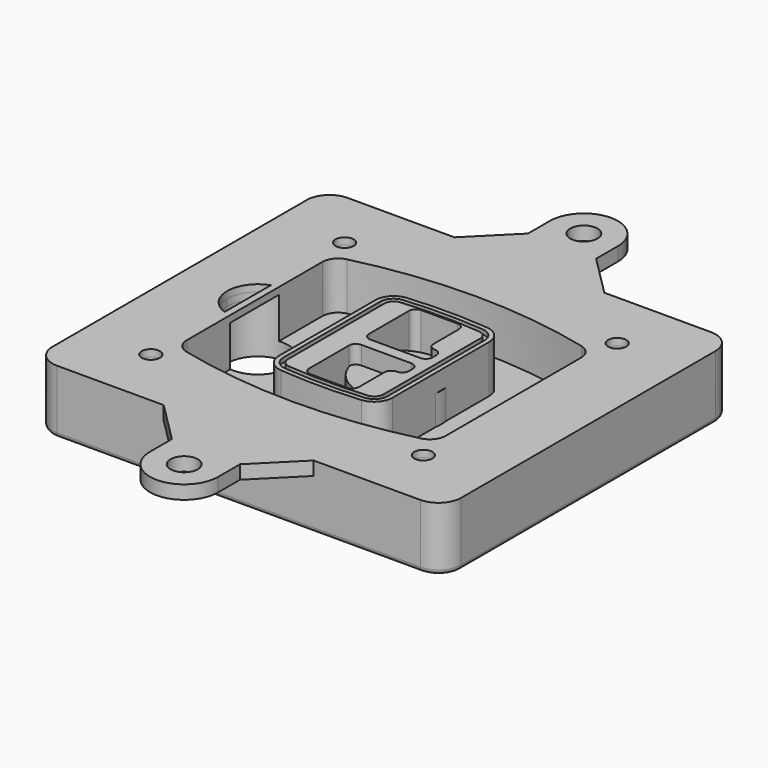
from build123d import *

# Parameters (mm, degrees)
F0_R      = 4
F1_DEPTH  = 25
F2_DEPTH  = 3
F3_DEPTH  = 18
F5_DEPTH  = 21
F6_DEPTH  = 2
F8_DEPTH  = 20
F9_DEPTH  = 16
F10_DEPTH = 25
F7_R      = 6
F7_R_2    = 4
F11_DEPTH = 6
F13_DEPTH = 9
F15_R     = 2
F16_R     = 6
F16_R_2   = 4
F17_DEPTH = 3


# Not quite as in the source:
# - a feature of the source that left no trace in its solid (it failed there, or was rolled back) is left out
# - a feature names something its author has since deleted; it is built from what else it names


with BuildPart() as f1:
    # F0 (on Top) → F1 (new body)
    with BuildSketch(Plane.XY):
        with BuildLine():
            ThreePointArc((-90, -70), (-87.0710678119, -77.0710678119), (-80, -80))
            Line((-80, -80), (80, -80))
            ThreePointArc((80, -80), (87.0710678119, -77.0710678119), (90, -70))
            Line((90, -70), (90, 70))
            ThreePointArc((90, 70), (87.0710678119, 77.0710678119), (80, 80))
            Line((80, 80), (-80, 80))
            ThreePointArc((-80, 80), (-87.0710678119, 77.0710678119), (-90, 70))
            Line((-90, 70), (-90, -70))
        make_face()
        with Locations((-60, -53.3333333333)):
            Circle(F0_R, mode=Mode.SUBTRACT)
        with Locations((60, -53.3333333333)):
            Circle(F0_R, mode=Mode.SUBTRACT)
        with Locations((-60, 53.3333333333)):
            Circle(F0_R, mode=Mode.SUBTRACT)
        with BuildLine():
            ThreePointArc((-64, 37.2990447398), (-61.0143011354, 45.9411029726), (-53.3306899286, 50.8970778549))
            ThreePointArc((-53.3306899286, 50.8970778549), (0, 57.3333333333), (53.3306899286, 50.8970778549))
            ThreePointArc((53.3306899286, 50.8970778549), (61.0143011354, 45.9411029726), (64, 37.2990447398))
            Line((64, 37.2990447398), (64, -37.2990447398))
            ThreePointArc((64, -37.2990447398), (61.0143011354, -45.9411029726), (53.3306899286, -50.8970778549))
            ThreePointArc((53.3306899286, -50.8970778549), (0, -57.3333333333), (-53.3306899286, -50.8970778549))
            ThreePointArc((-53.3306899286, -50.8970778549), (-61.0143011354, -45.9411029726), (-64, -37.2990447398))
            Line((-64, -37.2990447398), (-64, 37.2990447398))
        make_face(mode=Mode.SUBTRACT)
        with Locations((60, 53.3333333333)):
            Circle(F0_R, mode=Mode.SUBTRACT)
        with BuildLine():
            ThreePointArc((53.3306899286, 50.8970778549), (0, 57.3333333333), (-53.3306899286, 50.8970778549))
            ThreePointArc((-53.3306899286, 50.8970778549), (-61.0143011354, 45.9411029726), (-64, 37.2990447398))
            Line((-64, 37.2990447398), (-64, -37.2990447398))
            ThreePointArc((-64, -37.2990447398), (-61.0143011354, -45.9411029726), (-53.3306899286, -50.8970778549))
            ThreePointArc((-53.3306899286, -50.8970778549), (0, -57.3333333333), (53.3306899286, -50.8970778549))
            ThreePointArc((53.3306899286, -50.8970778549), (61.0143011354, -45.9411029726), (64, -37.2990447398))
            Line((64, -37.2990447398), (64, 37.2990447398))
            ThreePointArc((64, 37.2990447398), (61.0143011354, 45.9411029726), (53.3306899286, 50.8970778549))
        make_face()
        with BuildLine():
            Line((-60, -37.2990447398), (-60, 37.2990447398))
            ThreePointArc((-60, 37.2990447398), (-57.8673579538, 43.4719434775), (-52.3790642347, 47.0119255363))
            ThreePointArc((-52.3790642347, 47.0119255363), (0, 53.3333333333), (52.3790642347, 47.0119255363))
            ThreePointArc((52.3790642347, 47.0119255363), (57.8673579538, 43.4719434775), (60, 37.2990447398))
            Line((60, 37.2990447398), (60, -37.2990447398))
            ThreePointArc((60, -37.2990447398), (57.8673579538, -43.4719434775), (52.3790642347, -47.0119255363))
            ThreePointArc((52.3790642347, -47.0119255363), (0, -53.3333333333), (-52.3790642347, -47.0119255363))
            ThreePointArc((-52.3790642347, -47.0119255363), (-57.8673579538, -43.4719434775), (-60, -37.2990447398))
        make_face(mode=Mode.SUBTRACT)
        with BuildLine():
            ThreePointArc((-52.3790642347, 47.0119255363), (-57.8673579538, 43.4719434775), (-60, 37.2990447398))
            Line((-60, 37.2990447398), (-60, -37.2990447398))
            ThreePointArc((-60, -37.2990447398), (-57.8673579538, -43.4719434775), (-52.3790642347, -47.0119255363))
            ThreePointArc((-52.3790642347, -47.0119255363), (0, -53.3333333333), (52.3790642347, -47.0119255363))
            ThreePointArc((52.3790642347, -47.0119255363), (57.8673579538, -43.4719434775), (60, -37.2990447398))
            Line((60, -37.2990447398), (60, 37.2990447398))
            ThreePointArc((60, 37.2990447398), (57.8673579538, 43.4719434775), (52.3790642347, 47.0119255363))
            ThreePointArc((52.3790642347, 47.0119255363), (0, 53.3333333333), (-52.3790642347, 47.0119255363))
        make_face()
        with BuildLine():
            ThreePointArc((51.6653449643, 44.0980612973), (55.5071505677, 41.6200738562), (57, 37.2990447398))
            Line((57, 37.2990447398), (57, -37.2990447398))
            ThreePointArc((57, -37.2990447398), (55.5071505677, -41.6200738562), (51.6653449643, -44.0980612973))
            ThreePointArc((51.6653449643, -44.0980612973), (0, -50.3333333333), (-51.6653449643, -44.0980612973))
            ThreePointArc((-51.6653449643, -44.0980612973), (-55.5071505677, -41.6200738562), (-57, -37.2990447398))
            Line((-57, -37.2990447398), (-57, 37.2990447398))
            ThreePointArc((-57, 37.2990447398), (-55.5071505677, 41.6200738562), (-51.6653449643, 44.0980612973))
            ThreePointArc((-51.6653449643, 44.0980612973), (0, 50.3333333333), (51.6653449643, 44.0980612973))
        make_face(mode=Mode.SUBTRACT)
        with BuildLine():
            Line((57, -37.2990447398), (57, 37.2990447398))
            ThreePointArc((57, 37.2990447398), (55.5071505677, 41.6200738562), (51.6653449643, 44.0980612973))
            ThreePointArc((51.6653449643, 44.0980612973), (0, 50.3333333333), (-51.6653449643, 44.0980612973))
            ThreePointArc((-51.6653449643, 44.0980612973), (-55.5071505677, 41.6200738562), (-57, 37.2990447398))
            Line((-57, 37.2990447398), (-57, -37.2990447398))
            ThreePointArc((-57, -37.2990447398), (-55.5071505677, -41.6200738562), (-51.6653449643, -44.0980612973))
            ThreePointArc((-51.6653449643, -44.0980612973), (0, -50.3333333333), (51.6653449643, -44.0980612973))
            ThreePointArc((51.6653449643, -44.0980612973), (55.5071505677, -41.6200738562), (57, -37.2990447398))
        make_face()
    extrude(amount=-F1_DEPTH)

    # F0 (on Top) → F2 (join)
    with BuildSketch(Plane.XY):
        with BuildLine():
            ThreePointArc((-52.3790642347, 47.0119255363), (-57.8673579538, 43.4719434775), (-60, 37.2990447398))
            Line((-60, 37.2990447398), (-60, -37.2990447398))
            ThreePointArc((-60, -37.2990447398), (-57.8673579538, -43.4719434775), (-52.3790642347, -47.0119255363))
            ThreePointArc((-52.3790642347, -47.0119255363), (0, -53.3333333333), (52.3790642347, -47.0119255363))
            ThreePointArc((52.3790642347, -47.0119255363), (57.8673579538, -43.4719434775), (60, -37.2990447398))
            Line((60, -37.2990447398), (60, 37.2990447398))
            ThreePointArc((60, 37.2990447398), (57.8673579538, 43.4719434775), (52.3790642347, 47.0119255363))
            ThreePointArc((52.3790642347, 47.0119255363), (0, 53.3333333333), (-52.3790642347, 47.0119255363))
        make_face()
        with BuildLine():
            ThreePointArc((51.6653449643, 44.0980612973), (55.5071505677, 41.6200738562), (57, 37.2990447398))
            Line((57, 37.2990447398), (57, -37.2990447398))
            ThreePointArc((57, -37.2990447398), (55.5071505677, -41.6200738562), (51.6653449643, -44.0980612973))
            ThreePointArc((51.6653449643, -44.0980612973), (0, -50.3333333333), (-51.6653449643, -44.0980612973))
            ThreePointArc((-51.6653449643, -44.0980612973), (-55.5071505677, -41.6200738562), (-57, -37.2990447398))
            Line((-57, -37.2990447398), (-57, 37.2990447398))
            ThreePointArc((-57, 37.2990447398), (-55.5071505677, 41.6200738562), (-51.6653449643, 44.0980612973))
            ThreePointArc((-51.6653449643, 44.0980612973), (0, 50.3333333333), (51.6653449643, 44.0980612973))
        make_face(mode=Mode.SUBTRACT)
    extrude(amount=F2_DEPTH)

    # F0 (on Top) → F3 (cut)
    with BuildSketch(Plane.XY):
        with BuildLine():
            Line((57, -37.2990447398), (57, 37.2990447398))
            ThreePointArc((57, 37.2990447398), (55.5071505677, 41.6200738562), (51.6653449643, 44.0980612973))
            ThreePointArc((51.6653449643, 44.0980612973), (0, 50.3333333333), (-51.6653449643, 44.0980612973))
            ThreePointArc((-51.6653449643, 44.0980612973), (-55.5071505677, 41.6200738562), (-57, 37.2990447398))
            Line((-57, 37.2990447398), (-57, -37.2990447398))
            ThreePointArc((-57, -37.2990447398), (-55.5071505677, -41.6200738562), (-51.6653449643, -44.0980612973))
            ThreePointArc((-51.6653449643, -44.0980612973), (0, -50.3333333333), (51.6653449643, -44.0980612973))
            ThreePointArc((51.6653449643, -44.0980612973), (55.5071505677, -41.6200738562), (57, -37.2990447398))
        make_face()
    extrude(amount=-F3_DEPTH, mode=Mode.SUBTRACT)

    # F4 (on face) → F5 (join, through all)
    with BuildSketch(Plane.XY.offset(3)):
        with BuildLine():
            ThreePointArc((-25, -26.587695628), (-22.8992979869, -31.9912392117), (-17.7004291845, -34.5569740744))
            ThreePointArc((-17.7004291845, -34.5569740744), (0, -35.3333333333), (17.7004291845, -34.5569740744))
            ThreePointArc((17.7004291845, -34.5569740744), (22.8992979869, -31.9912392117), (25, -26.587695628))
            Line((25, -26.587695628), (25, 26.587695628))
            ThreePointArc((25, 26.587695628), (22.8992979869, 31.9912392117), (17.7004291845, 34.5569740744))
            ThreePointArc((17.7004291845, 34.5569740744), (0, 35.3333333333), (-17.7004291845, 34.5569740744))
            ThreePointArc((-17.7004291845, 34.5569740744), (-22.8992979869, 31.9912392117), (-25, 26.587695628))
            Line((-25, 26.587695628), (-25, -26.587695628))
        make_face()
        with BuildLine():
            ThreePointArc((17.5253218884, 32.5646544628), (21.4244734902, 30.6403533158), (23, 26.587695628))
            Line((23, 26.587695628), (23, -26.587695628))
            ThreePointArc((23, -26.587695628), (21.4244734902, -30.6403533158), (17.5253218884, -32.5646544628))
            ThreePointArc((17.5253218884, -32.5646544628), (0, -33.3333333333), (-17.5253218884, -32.5646544628))
            ThreePointArc((-17.5253218884, -32.5646544628), (-21.4244734902, -30.6403533158), (-23, -26.587695628))
            Line((-23, -26.587695628), (-23, 26.587695628))
            ThreePointArc((-23, 26.587695628), (-21.4244734902, 30.6403533158), (-17.5253218884, 32.5646544628))
            ThreePointArc((-17.5253218884, 32.5646544628), (0, 33.3333333333), (17.5253218884, 32.5646544628))
        make_face(mode=Mode.SUBTRACT)
        with BuildLine():
            Line((23, -26.587695628), (23, 26.587695628))
            ThreePointArc((23, 26.587695628), (21.4244734902, 30.6403533158), (17.5253218884, 32.5646544628))
            ThreePointArc((17.5253218884, 32.5646544628), (0, 33.3333333333), (-17.5253218884, 32.5646544628))
            ThreePointArc((-17.5253218884, 32.5646544628), (-21.4244734902, 30.6403533158), (-23, 26.587695628))
            Line((-23, 26.587695628), (-23, -26.587695628))
            ThreePointArc((-23, -26.587695628), (-21.4244734902, -30.6403533158), (-17.5253218884, -32.5646544628))
            ThreePointArc((-17.5253218884, -32.5646544628), (0, -33.3333333333), (17.5253218884, -32.5646544628))
            ThreePointArc((17.5253218884, -32.5646544628), (21.4244734902, -30.6403533158), (23, -26.587695628))
        make_face()
        with BuildLine():
            ThreePointArc((17.3502145923, 30.5723348512), (19.9496489934, 29.2894674198), (21, 26.587695628))
            Line((21, 26.587695628), (21, -26.587695628))
            ThreePointArc((21, -26.587695628), (19.9496489934, -29.2894674198), (17.3502145923, -30.5723348512))
            ThreePointArc((17.3502145923, -30.5723348512), (0, -31.3333333333), (-17.3502145923, -30.5723348512))
            ThreePointArc((-17.3502145923, -30.5723348512), (-19.9496489934, -29.2894674198), (-21, -26.587695628))
            Line((-21, -26.587695628), (-21, 26.587695628))
            ThreePointArc((-21, 26.587695628), (-19.9496489934, 29.2894674198), (-17.3502145923, 30.5723348512))
            ThreePointArc((-17.3502145923, 30.5723348512), (0, 31.3333333333), (17.3502145923, 30.5723348512))
        make_face(mode=Mode.SUBTRACT)
        with BuildLine():
            Line((21, -26.587695628), (21, 26.587695628))
            ThreePointArc((21, 26.587695628), (19.9496489934, 29.2894674198), (17.3502145923, 30.5723348512))
            ThreePointArc((17.3502145923, 30.5723348512), (0, 31.3333333333), (-17.3502145923, 30.5723348512))
            ThreePointArc((-17.3502145923, 30.5723348512), (-19.9496489934, 29.2894674198), (-21, 26.587695628))
            Line((-21, 26.587695628), (-21, -26.587695628))
            ThreePointArc((-21, -26.587695628), (-19.9496489934, -29.2894674198), (-17.3502145923, -30.5723348512))
            ThreePointArc((-17.3502145923, -30.5723348512), (0, -31.3333333333), (17.3502145923, -30.5723348512))
            ThreePointArc((17.3502145923, -30.5723348512), (19.9496489934, -29.2894674198), (21, -26.587695628))
        make_face()
        with BuildLine():
            Line((-8, -2.5), (14, -2.5))
            ThreePointArc((14, -2.5), (16.1213203436, -3.3786796564), (17, -5.5))
            Line((17, -5.5), (17, -7.5))
            ThreePointArc((17, -7.5), (16.1213203436, -9.6213203436), (14, -10.5))
            ThreePointArc((14, -10.5), (11.8786796564, -11.3786796564), (11, -13.5))
            Line((11, -13.5), (11, -27.5))
            ThreePointArc((11, -27.5), (10.1213203436, -29.6213203436), (8, -30.5))
            Line((8, -30.5), (-8, -30.5))
            ThreePointArc((-8, -30.5), (-10.1213203436, -29.6213203436), (-11, -27.5))
            Line((-11, -27.5), (-11, -5.5))
            ThreePointArc((-11, -5.5), (-10.1213203436, -3.3786796564), (-8, -2.5))
        make_face(mode=Mode.SUBTRACT)
        with BuildLine():
            ThreePointArc((-8, 2.5), (-10.1213203436, 3.3786796564), (-11, 5.5))
            Line((-11, 5.5), (-11, 27.5))
            ThreePointArc((-11, 27.5), (-10.1213203436, 29.6213203436), (-8, 30.5))
            Line((-8, 30.5), (8, 30.5))
            ThreePointArc((8, 30.5), (10.1213203436, 29.6213203436), (11, 27.5))
            Line((11, 27.5), (11, 13.5))
            ThreePointArc((11, 13.5), (11.8786796564, 11.3786796564), (14, 10.5))
            ThreePointArc((14, 10.5), (16.1213203436, 9.6213203436), (17, 7.5))
            Line((17, 7.5), (17, 5.5))
            ThreePointArc((17, 5.5), (16.1213203436, 3.3786796564), (14, 2.5))
            Line((14, 2.5), (-8, 2.5))
        make_face(mode=Mode.SUBTRACT)
    extrude(amount=-F5_DEPTH)

    # F4 (on face) → F6 (cut)
    with BuildSketch(Plane.XY.offset(3)):
        with BuildLine():
            Line((23, -26.587695628), (23, 26.587695628))
            ThreePointArc((23, 26.587695628), (21.4244734902, 30.6403533158), (17.5253218884, 32.5646544628))
            ThreePointArc((17.5253218884, 32.5646544628), (0, 33.3333333333), (-17.5253218884, 32.5646544628))
            ThreePointArc((-17.5253218884, 32.5646544628), (-21.4244734902, 30.6403533158), (-23, 26.587695628))
            Line((-23, 26.587695628), (-23, -26.587695628))
            ThreePointArc((-23, -26.587695628), (-21.4244734902, -30.6403533158), (-17.5253218884, -32.5646544628))
            ThreePointArc((-17.5253218884, -32.5646544628), (0, -33.3333333333), (17.5253218884, -32.5646544628))
            ThreePointArc((17.5253218884, -32.5646544628), (21.4244734902, -30.6403533158), (23, -26.587695628))
        make_face()
        with BuildLine():
            ThreePointArc((17.3502145923, 30.5723348512), (19.9496489934, 29.2894674198), (21, 26.587695628))
            Line((21, 26.587695628), (21, -26.587695628))
            ThreePointArc((21, -26.587695628), (19.9496489934, -29.2894674198), (17.3502145923, -30.5723348512))
            ThreePointArc((17.3502145923, -30.5723348512), (0, -31.3333333333), (-17.3502145923, -30.5723348512))
            ThreePointArc((-17.3502145923, -30.5723348512), (-19.9496489934, -29.2894674198), (-21, -26.587695628))
            Line((-21, -26.587695628), (-21, 26.587695628))
            ThreePointArc((-21, 26.587695628), (-19.9496489934, 29.2894674198), (-17.3502145923, 30.5723348512))
            ThreePointArc((-17.3502145923, 30.5723348512), (0, 31.3333333333), (17.3502145923, 30.5723348512))
        make_face(mode=Mode.SUBTRACT)
    extrude(amount=-F6_DEPTH, mode=Mode.SUBTRACT)

    # F7 (on face) → F8 (join)
    with BuildSketch(Plane(origin=(0, 0, -25), x_dir=(1, 0, 0), z_dir=(0, 0, -1))):
        with BuildLine():
            ThreePointArc((-6.71157564, 0), (6.7567035675, 13.4682792075), (20.224982775, 0))
            Line((20.224982775, 0), (25.224982775, 0))
            ThreePointArc((25.224982775, 0), (6.7567035675, 18.4682792075), (-11.71157564, 0))
            Line((-11.71157564, 0), (-6.71157564, 0))
        make_face()
        with BuildLine():
            Line((-6.71157564, 0), (20.224982775, 0))
            ThreePointArc((20.224982775, 0), (6.7567035675, 13.4682792075), (-6.71157564, 0))
        make_face()
        with BuildLine():
            ThreePointArc((-6.71157564, 0), (6.7567035675, -13.4682792075), (20.224982775, 0))
            Line((20.224982775, 0), (-6.71157564, 0))
        make_face()
        with BuildLine():
            Line((25.224982775, 0), (20.224982775, 0))
            ThreePointArc((20.224982775, 0), (6.7567035675, -13.4682792075), (-6.71157564, 0))
            Line((-6.71157564, 0), (-11.71157564, 0))
            ThreePointArc((-11.71157564, 0), (6.7567035675, -18.4682792075), (25.224982775, 0))
        make_face()
    extrude(amount=-F8_DEPTH)

    # F7 (on face) → F9 (cut)
    with BuildSketch(Plane(origin=(0, 0, -25), x_dir=(1, 0, 0), z_dir=(0, 0, -1))):
        with BuildLine():
            Line((-6.71157564, 0), (20.224982775, 0))
            ThreePointArc((20.224982775, 0), (6.7567035675, 13.4682792075), (-6.71157564, 0))
        make_face()
        with BuildLine():
            ThreePointArc((-6.71157564, 0), (6.7567035675, -13.4682792075), (20.224982775, 0))
            Line((20.224982775, 0), (-6.71157564, 0))
        make_face()
    extrude(amount=-F9_DEPTH, mode=Mode.SUBTRACT)

    # F7 (on face) → F10 (cut)
    with BuildSketch(Plane(origin=(0, 0, -25), x_dir=(1, 0, 0), z_dir=(0, 0, -1))):
        with BuildLine():
            Line((-69.0318229325, 0), (-42.0952645175, 0))
            ThreePointArc((-42.0952645175, 0), (-55.563543725, 13.4682792075), (-69.0318229325, 0))
        make_face()
        with BuildLine():
            ThreePointArc((-69.0318229325, 0), (-55.563543725, -13.4682792075), (-42.0952645175, 0))
            Line((-42.0952645175, 0), (-69.0318229325, 0))
        make_face()
    extrude(amount=-F10_DEPTH, mode=Mode.SUBTRACT)

    # F7 (on face) → F11 (cut)
    with BuildSketch(Plane(origin=(0, 0, -25), x_dir=(1, 0, 0), z_dir=(0, 0, -1))):
        with Locations((60, -53.3333333333)):
            Circle(F7_R)
        with Locations((60, -53.3333333333)):
            Circle(F7_R_2, mode=Mode.SUBTRACT)
        with Locations((-60, -53.3333333333)):
            Circle(F7_R)
        with Locations((-60, -53.3333333333)):
            Circle(F7_R_2, mode=Mode.SUBTRACT)
        with Locations((-60, 53.3333333333)):
            Circle(F7_R)
        with Locations((-60, 53.3333333333)):
            Circle(F7_R_2, mode=Mode.SUBTRACT)
        with Locations((60, 53.3333333333)):
            Circle(F7_R)
        with Locations((60, 53.3333333333)):
            Circle(F7_R_2, mode=Mode.SUBTRACT)
    extrude(amount=-F11_DEPTH, mode=Mode.SUBTRACT)

    # F12 (on face) → F13 (cut, through all)
    with BuildSketch(Plane(origin=(0, 0, -9), x_dir=(1, 0, 0), z_dir=(0, 0, -1))):
        with BuildLine():
            ThreePointArc((20.224982775, 0), (20.1663399806, 1.2554664788), (19.9909222755, 2.5))
            Line((19.9909222755, 2.5), (14, 2.5))
            ThreePointArc((14, 2.5), (16.1213203436, 3.3786796564), (17, 5.5))
            Line((17, 5.5), (17, 7.5))
            ThreePointArc((17, 7.5), (16.1213203436, 9.6213203436), (14, 10.5))
            ThreePointArc((14, 10.5), (12.1627255951, 11.1284134507), (11.0951631559, 12.750384826))
            ThreePointArc((11.0951631559, 12.750384826), (11.0476113807, 12.7664660322), (11, 12.7823698976))
            Line((11, 12.7823698976), (11, -12.7823698976))
            ThreePointArc((11, -12.7823698976), (11.0476113807, -12.7664660322), (11.0951631559, -12.750384826))
            ThreePointArc((11.0951631559, -12.750384826), (12.1627255951, -11.1284134507), (14, -10.5))
            ThreePointArc((14, -10.5), (16.1213203436, -9.6213203436), (17, -7.5))
            Line((17, -7.5), (17, -5.5))
            ThreePointArc((17, -5.5), (16.1213203436, -3.3786796564), (14, -2.5))
            Line((14, -2.5), (19.9909222755, -2.5))
            ThreePointArc((19.9909222755, -2.5), (20.1663399806, -1.2554664788), (20.224982775, 0))
        make_face()
    extrude(amount=F13_DEPTH, mode=Mode.SUBTRACT)

    # F15
    f15_edges = [f1.edges().sort_by_distance(p)[0] for p in [
        (0, -80, -25),
        (-87.071068, -77.071068, -25),
        (-90, 0, -25),
        (-87.071068, 77.071068, -25),
        (87.071068, -77.071068, -25),
        (0, 80, -25),
        (90, 0, -25),
        (87.071068, 77.071068, -25),
    ]]
    fillet(f15_edges, radius=F15_R)

    # F16 (on face) → F17 (join, symmetric)
    with BuildSketch(Plane.XY):
        with BuildLine():
            Line((-33, 80), (33, 80))
            Line((33, 80), (15, 98))
            Line((15, 98), (15, 110))
            ThreePointArc((15, 110), (0, 125), (-15, 110))
            Line((-15, 110), (-15, 98))
            Line((-15, 98), (-33, 80))
        make_face()
        with Locations((0, 110)):
            Circle(F16_R, mode=Mode.SUBTRACT)
        with BuildLine():
            Line((90, -70), (90, 70))
            ThreePointArc((90, 70), (87.0710678119, 77.0710678119), (80, 80))
            Line((80, 80), (33, 80))
            Line((33, 80), (-33, 80))
            Line((-33, 80), (-80, 80))
            ThreePointArc((-80, 80), (-87.0710678119, 77.0710678119), (-90, 70))
            Line((-90, 70), (-90, -70))
            ThreePointArc((-90, -70), (-87.0710678119, -77.0710678119), (-80, -80))
            Line((-80, -80), (-33, -80))
            Line((-33, -80), (33, -80))
            Line((33, -80), (80, -80))
            ThreePointArc((80, -80), (87.0710678119, -77.0710678119), (90, -70))
        make_face()
        with Locations((-60, -53.3333333333)):
            Circle(F16_R_2, mode=Mode.SUBTRACT)
        with Locations((60, -53.3333333333)):
            Circle(F16_R_2, mode=Mode.SUBTRACT)
        with Locations((-60, 53.3333333333)):
            Circle(F16_R_2, mode=Mode.SUBTRACT)
        with BuildLine():
            ThreePointArc((-52.3790642347, 47.0119255363), (0, 53.3333333333), (52.3790642347, 47.0119255363))
            ThreePointArc((52.3790642347, 47.0119255363), (57.8673579538, 43.4719434775), (60, 37.2990447398))
            Line((60, 37.2990447398), (60, -37.2990447398))
            ThreePointArc((60, -37.2990447398), (57.8673579538, -43.4719434775), (52.3790642347, -47.0119255363))
            ThreePointArc((52.3790642347, -47.0119255363), (0, -53.3333333333), (-52.3790642347, -47.0119255363))
            ThreePointArc((-52.3790642347, -47.0119255363), (-57.8673579538, -43.4719434775), (-60, -37.2990447398))
            Line((-60, -37.2990447398), (-60, -12.7166190685))
            ThreePointArc((-60, -12.7166190685), (-66.5441169481, -7.798817635), (-69.0318229325, 0))
            ThreePointArc((-69.0318229325, 0), (-66.5441169481, 7.798817635), (-60, 12.7166190685))
            Line((-60, 12.7166190685), (-60, 37.2990447398))
            ThreePointArc((-60, 37.2990447398), (-57.8673579538, 43.4719434775), (-52.3790642347, 47.0119255363))
        make_face(mode=Mode.SUBTRACT)
        with Locations((60, 53.3333333333)):
            Circle(F16_R_2, mode=Mode.SUBTRACT)
        with BuildLine():
            Line((15, -98), (33, -80))
            Line((33, -80), (-33, -80))
            Line((-33, -80), (-15, -98))
            Line((-15, -98), (-15, -110))
            ThreePointArc((-15, -110), (0, -125), (15, -110))
            Line((15, -110), (15, -98))
        make_face()
        with Locations((0, -110)):
            Circle(F16_R, mode=Mode.SUBTRACT)
    extrude(amount=F17_DEPTH, both=True)


solid = f1.part
